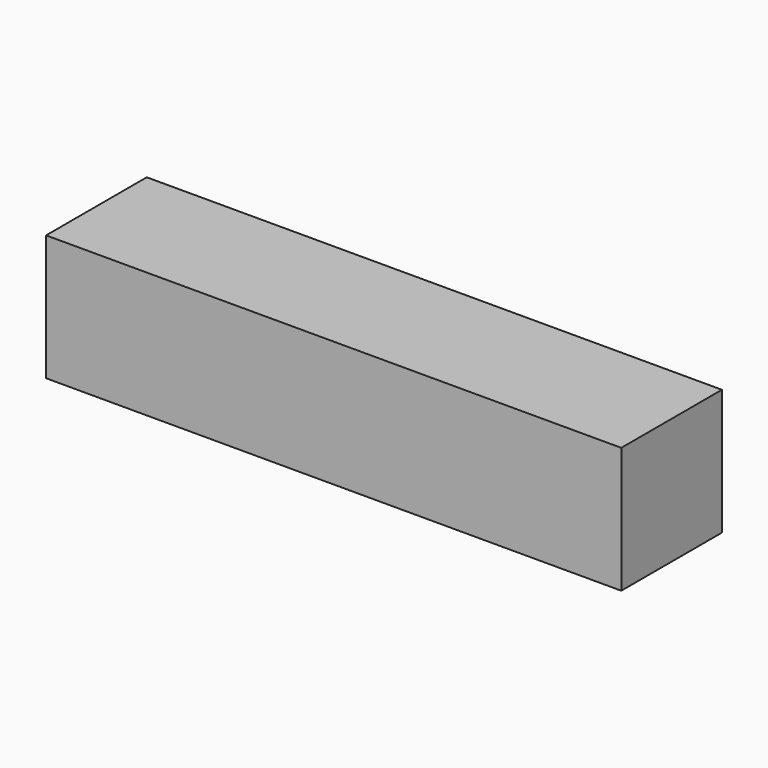
from build123d import *

# Parameters (mm, degrees)
F0_W        = 228.6
F0_H        = 50
F1_DEPTH    = 50
F3_DEPTH    = 48
F4_R        = 11
F5_DEPTH    = 9
F7_DEPTH    = 15
F8_T2_ANGLE = 343.7894292622


# Not quite as in the source:
# - a fillet or chamfer that OpenCascade refuses, or shapes differently, is made with other operations: its cross-section is extruded or revolved along the edge and cut away or added


with BuildPart() as f1:
    # F0 (on Front) → F1 (new body)
    with BuildSketch(Plane.XZ):
        Rectangle(F0_W, F0_H)
    extrude(amount=F1_DEPTH)

    # F2 (on face) → F3 (cut)
    with BuildSketch(Plane(origin=(0, 0, 0), x_dir=(-1, 0, 0), z_dir=(0, 1, 0))):
        Polygon((-106.0638769388, 21.0001030612), (-110.06398, 17), (-110.06398, -17), (-106.0638769388, -21.0001030612), (-72.0638769388, -21.0001030612), (-68.0637738777, -17), (-68.0637738777, 17), (-72.0638769388, 21.0001030612), align=None)
    extrude(amount=-F3_DEPTH, mode=Mode.SUBTRACT)

    # F4 (on face) → F5 (cut)
    with BuildSketch(Plane(origin=(0, 0, 0), x_dir=(-1, 0, 0), z_dir=(0, 1, 0))):
        with Locations((89.3, 0)):
            Circle(F4_R)
    extrude(amount=-F5_DEPTH, mode=Mode.SUBTRACT)

    # F6 (on face) → F7 (cut)
    with BuildSketch(Plane(origin=(0, -9, 0), x_dir=(-1, 0, 0), z_dir=(0, 1, 0))):
        with BuildLine():
            Line((90.8, 2), (87.8, 2))
            ThreePointArc((87.8, 2), (89.3, -2.5), (90.8, 2))
        make_face()
    extrude(amount=-F7_DEPTH, mode=Mode.SUBTRACT)

    # F8: fillet of radius 0.5 on 1 edges, made by hand

    # F8_s1 → F8_t2 (revolve)
    with BuildSketch(Plane(origin=(-87.5248141005, 0, 12.4648632504), x_dir=(0, 1, 0), z_dir=(-0.9900106558, 0, 0.1409925581))):
        with BuildLine():
            ThreePointArc((-23.5, 10.0906354418), (-23.8535533906, 10.2370820512), (-24, 10.5906354418))
            Line((-24, 10.5906354418), (-24, 10.0906354418))
            Line((-24, 10.0906354418), (-23.5, 10.0906354418))
        make_face()
    revolve(axis=Axis((-89.3, -24, 0), (0, 1, 0)), revolution_arc=F8_T2_ANGLE)


solid = f1.part
